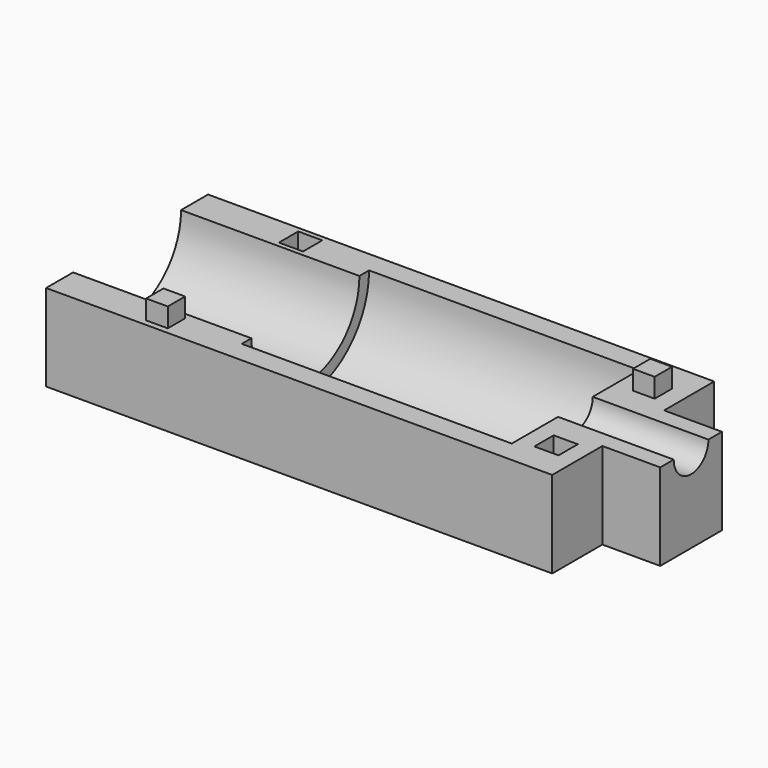
from build123d import *

# Parameters (mm, degrees)
F0_W      = 80
F0_H      = 42
F1_DEPTH  = 22
F3_DEPTH  = 80
F4_DEPTH  = 2
F6_DEPTH  = 22
F7_DEPTH  = 28
F8_DEPTH  = 15
F9_DEPTH  = 2
F10_DEPTH = 10
F11_W     = 5
F11_H     = 5
F12_DEPTH = 4
F11_W_2   = 4.5
F11_H_2   = 4.5
F13_DEPTH = 4
F14_DEPTH = 12
F15_DEPTH = 4
F16_W     = 13
F16_H     = 18
F17_DEPTH = 12


# Not quite as in the source:
# - a feature names something its author has since deleted; it is built from what else it names


with BuildPart() as f1:
    # F0 (on Top) → F1 (new body)
    with BuildSketch(Plane.XY):
        Rectangle(F0_W, F0_H)
    extrude(amount=F1_DEPTH)

    # F2 (on face) → F3 (cut)
    with BuildSketch(Plane.YZ.offset(40)):
        with BuildLine():
            ThreePointArc((-16.5, 22), (0, 5.5), (16.5, 22))
            Line((16.5, 22), (14, 22))
            ThreePointArc((14, 22), (0, 8), (-14, 22))
            Line((-14, 22), (-16.5, 22))
        make_face()
        with BuildLine():
            ThreePointArc((-14, 22), (0, 8), (14, 22))
            Line((14, 22), (4.5, 22))
            ThreePointArc((4.5, 22), (0, 17.5), (-4.5, 22))
            Line((-4.5, 22), (-14, 22))
        make_face()
        with BuildLine():
            ThreePointArc((-4.5, 22), (0, 17.5), (4.5, 22))
            Line((4.5, 22), (-4.5, 22))
        make_face()
    extrude(amount=-F3_DEPTH, mode=Mode.SUBTRACT)

    # F2 (on face) → F4 (join)
    with BuildSketch(Plane.YZ.offset(40)):
        with BuildLine():
            ThreePointArc((-16.5, 22), (0, 5.5), (16.5, 22))
            Line((16.5, 22), (14, 22))
            ThreePointArc((14, 22), (0, 8), (-14, 22))
            Line((-14, 22), (-16.5, 22))
        make_face()
    extrude(amount=-F4_DEPTH)



with BuildPart() as f6:
    # F5 (on face) → F6 (new body)
    with BuildSketch(Plane(origin=(-40, 0, 0), x_dir=(0, -1, 0), z_dir=(-1, 0, 0))):
        with BuildLine():
            Line((-14, 22), (14, 22))
            ThreePointArc((14, 22), (0, 36), (-14, 22))
        make_face()
    extrude(amount=-F6_DEPTH)


with BuildPart() as f1_1:
    add(f1.part)

    add(f6.part)  # F6#2 merges F6
    # F5 (on face) → F6, piece 2 (join)
    with BuildSketch(Plane(origin=(-40, 0, 0), x_dir=(0, -1, 0), z_dir=(-1, 0, 0))):
        with BuildLine():
            Line((16.5, 22), (14, 22))
            ThreePointArc((14, 22), (0, 8), (-14, 22))
            Line((-14, 22), (-16.5, 22))
            ThreePointArc((-16.5, 22), (0, 5.5), (16.5, 22))
        make_face()
        with BuildLine():
            Line((21, 22), (16.5, 22))
            ThreePointArc((16.5, 22), (0, 5.5), (-16.5, 22))
            Line((-16.5, 22), (-21, 22))
            Line((-21, 22), (-21, 0))
            Line((-21, 0), (21, 0))
            Line((21, 0), (21, 22))
        make_face()
    extrude(amount=-F6_DEPTH)

    # F5 (on face) → F7 (cut)
    with BuildSketch(Plane(origin=(-40, 0, 0), x_dir=(0, -1, 0), z_dir=(-1, 0, 0))):
        with BuildLine():
            Line((-14, 22), (14, 22))
            ThreePointArc((14, 22), (0, 36), (-14, 22))
        make_face()
    extrude(amount=-F7_DEPTH, mode=Mode.SUBTRACT)

    # F8 (add): a face of the model
    f8_faces = [f1_1.faces().sort_by_distance(p)[0] for p in [
        (-40, 0, 0.4741307836),
    ]]
    extrude(f8_faces, amount=F8_DEPTH)

    # F2 (on face) → F9 (join)
    with BuildSketch(Plane.YZ.offset(40)):
        with BuildLine():
            ThreePointArc((-14, 22), (0, 8), (14, 22))
            Line((14, 22), (4.5, 22))
            ThreePointArc((4.5, 22), (0, 17.5), (-4.5, 22))
            Line((-4.5, 22), (-14, 22))
        make_face()
    extrude(amount=-F9_DEPTH)

    # F10 (add): a face of the model
    f10_faces = [f1_1.faces().sort_by_distance(p)[0] for p in [
        (40, 0, 10.6759160757),
    ]]
    extrude(f10_faces, amount=F10_DEPTH)

    # F11 (on face) → F12 (cut)
    with BuildSketch(Plane.XY.offset(22)):
        with Locations((-33, 17.5)):
            Rectangle(F11_W, F11_H)
        with Locations((44, -12.5)):
            Rectangle(F11_W, F11_H)
    extrude(amount=-F12_DEPTH, mode=Mode.SUBTRACT)

    # F11 (on face) → F13 (join)
    with BuildSketch(Plane.XY.offset(22)):
        with Locations((-33, -17.5)):
            Rectangle(F11_W_2, F11_H_2)
        with Locations((44, 12.5)):
            Rectangle(F11_W_2, F11_H_2)
    extrude(amount=F13_DEPTH)

    # F14 (add): a face of the model
    f14_faces = [f1_1.faces().sort_by_distance(p)[0] for p in [
        (50, 0, 10.6759160757),
    ]]
    extrude(f14_faces, amount=F14_DEPTH)

    # F15 (cut): a face of the model
    f15_faces = [f1_1.faces().sort_by_distance(p)[0] for p in [
        (3.5, 0, 0),
    ]]
    extrude(f15_faces, amount=-F15_DEPTH, mode=Mode.SUBTRACT)

    # F16 (on face) → F17 (cut)
    with BuildSketch(Plane.YZ.offset(62)):
        with Locations((-14.5, 13)):
            Rectangle(F16_W, F16_H)
        with Locations((14.5, 13)):
            Rectangle(F16_W, F16_H)
    extrude(amount=-F17_DEPTH, mode=Mode.SUBTRACT)


solid = f1_1.part
